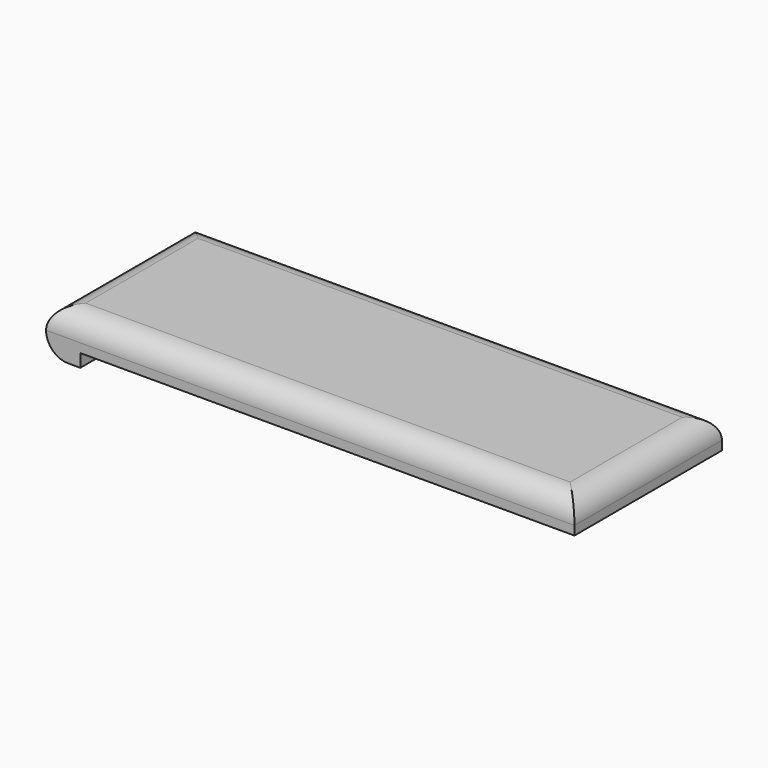
from build123d import *

# Parameters (mm, degrees)
F0_W     = 120
F0_H     = 41.8604637527
F1_DEPTH = 10
F2_W     = 112.2293550894
F2_H     = 2.9544678982
F3_DEPTH = 73.9
F4_R     = 4.99999


# Not quite as in the source:
# - a fillet or chamfer is up to 0.001 mm smaller than in the source, because OpenCascade refuses the exact size


with BuildPart() as f1:
    # F0 (on Top) → F1 (new body)
    with BuildSketch(Plane.XY):
        with Locations((-4.2187506333, 10.1562498603)):
            Rectangle(F0_W, F0_H)
    extrude(amount=F1_DEPTH)

    # F2 (on face) → F3 (cut)
    with BuildSketch(Plane.XZ.offset(10.773982016)):
        with Locations((-0.333428178, 1.4772339491)):
            Rectangle(F2_W, F2_H)
    extrude(amount=-F3_DEPTH, mode=Mode.SUBTRACT)

    # F4 (radius 5 in the source; OpenCascade refuses exactly that, so slightly less here)
    f4_edges = [f1.edges().sort_by_distance(p)[0] for p in [
        (-64.218751, 10.15625, 10),
        (-4.218751, 31.086482, 10),
        (-4.218751, -10.773982, 10),
        (55.781249, 10.15625, 10),
        (-64.218751, 10.15625, 0),
    ]]
    fillet(f4_edges, radius=F4_R)


solid = f1.part
